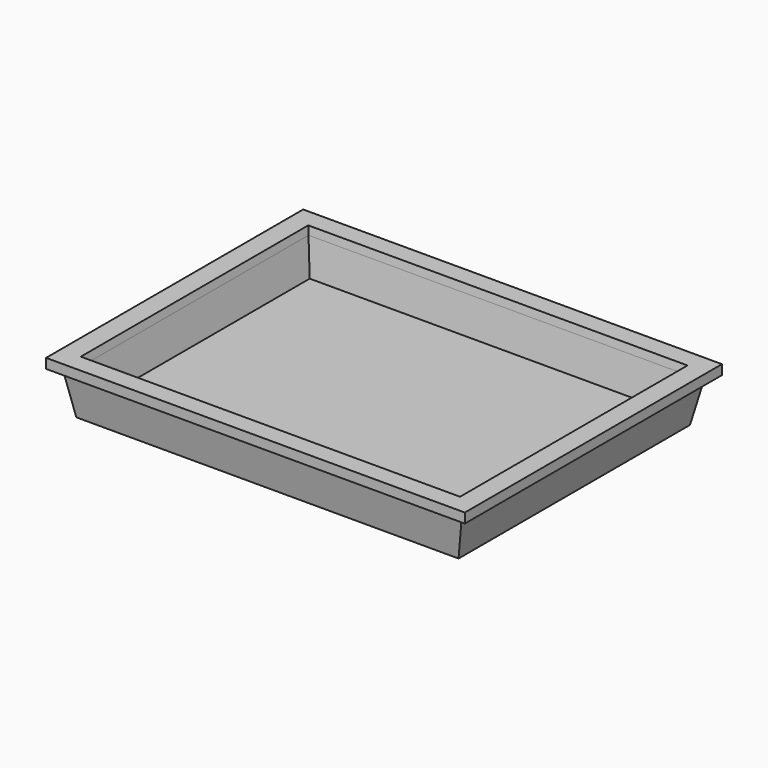
from build123d import *

# Parameters (mm, degrees)
F0_W          = 645
F0_H          = 495
F1_DEPTH      = 82
F3_DEPTH      = 322.501
F3_DEPTH_BACK = 495
F5_DEPTH      = 365
F5_DEPTH_BACK = 341
F6_T          = 18
F6_T3_DEPTH   = 505.2074342574
F6_T5_DEPTH   = 651


# Not quite as in the source:
# - a shell that OpenCascade refuses in one call is made with other operations: the cavity is built on its own and cut out


with BuildPart() as f1:
    # F0 (on Top) → F1 (new body)
    with BuildSketch(Plane.XY):
        Rectangle(F0_W, F0_H)
    extrude(amount=-F1_DEPTH)

    # F2 (on Right) → F3 (cut, two sides)
    with BuildSketch(Plane.YZ) as f3_sk:
        Polygon((-277.5, -15), (-277.5, -112), (-217.5, -112), (-234.6037171287, -15), align=None)
        Polygon((277.5, -15), (234.6037171287, -15), (217.5, -112), (277.5, -112), align=None)
    extrude(amount=F3_DEPTH, mode=Mode.SUBTRACT)
    extrude(f3_sk.sketch, amount=-F3_DEPTH_BACK, mode=Mode.SUBTRACT)

    # F4 (on Front) → F5 (cut, two sides)
    with BuildSketch(Plane.XZ) as f5_sk:
        Polygon((-337.5, -15), (-337.5, -185.1384545885), (-277.5, -185.1384545885), (-307.5, -15), align=None)
        Polygon((337.5, -15), (307.5, -15), (277.5415446769, -154.3605614963), (337.5, -156.5929672103), align=None)
    extrude(amount=F5_DEPTH, mode=Mode.SUBTRACT)
    extrude(f5_sk.sketch, amount=-F5_DEPTH_BACK, mode=Mode.SUBTRACT)

    # F6: shell of thickness 18, made by hand


with BuildPart() as f6_core1:
    # F6_t2: copy of F1
    add(f1.part)

    # the walls: a layer under each face that stays
    f6_faces = [f6_core1.faces().sort_by_distance(p)[0] for p in [
        (-322.5, 0, -7.5),
        (0, -247.5, -7.5),
        (322.5, 0, -7.5),
        (314.537037037, -170.15625, -15),
        (0, 228.696763275, -48.5),
        (-1.2945688909, 0, -82),
        (300.2984772553, 0, -48.5),
        (0, -228.696763275, -48.5),
        (-301.5930461463, 0, -48.5),
        (0, 247.5, -7.5),
    ]]
    thicken(f6_faces, amount=-F6_T, mode=Mode.SUBTRACT)

    # F6_s4 → F6_t3 (cut)
    with BuildSketch(Plane.XZ.offset(-252.6037171287)):
        Polygon((-307.6772653955, -15.211256672), (-307.5, 3), (-292.3962066388, 3), (-289.7734604458, -11.874332802), align=None)
        Polygon((307.6759796954, -15.2178305009), (307.5, 3), (292.9582599542, 3), (289.902030457, -11.2169499127), align=None)
    extrude(amount=F6_T3_DEPTH, mode=Mode.SUBTRACT)

    # F6_s6 → F6_t5 (cut)
    with BuildSketch(Plane.YZ.offset(-325.5)):
        Polygon((-234.7809825243, -15.211256672), (-234.6037171287, 3), (-219.4999237675, 3), (-216.8771775745, -11.874332802), align=None)
        Polygon((234.7809825243, -15.211256672), (234.6037171287, 3), (219.4999237675, 3), (216.8771775745, -11.874332802), align=None)
    extrude(amount=F6_T5_DEPTH, mode=Mode.SUBTRACT)


with BuildPart() as f1_1:
    add(f1.part)

    # what is left inside the walls is the cavity
    f6_cavity = [f6_core1.part.solids().sort_by_distance(p)[0] for p in [
        (0.223061, -72.990314, -0.18),
    ]]
    add(f6_cavity, mode=Mode.SUBTRACT)


solid = f1_1.part
